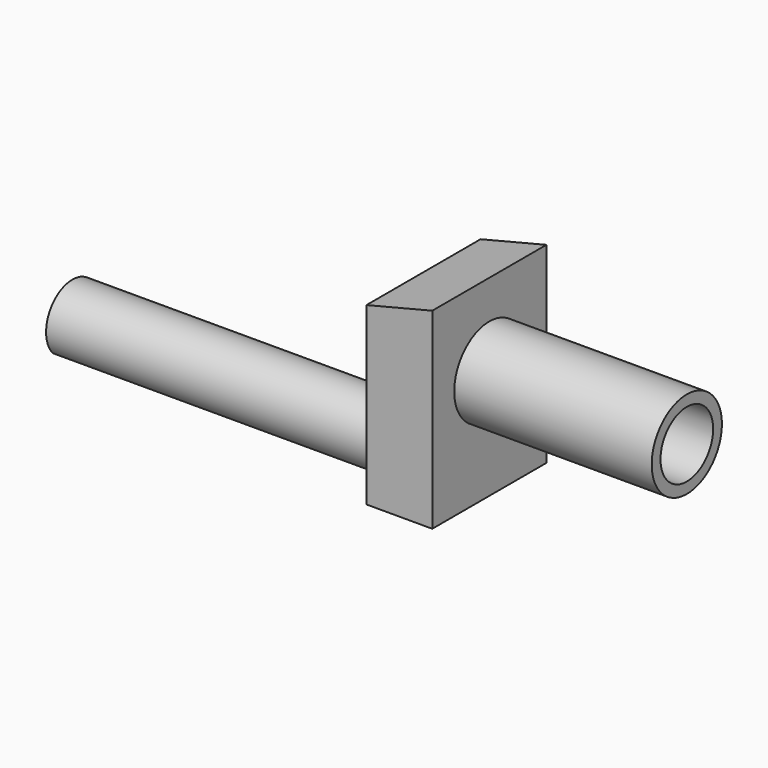
from build123d import *

# Parameters (mm, degrees)
F1_DEPTH  = 20.6375
F2_R      = 9.525
F3_DEPTH  = 50.8
F5_DEPTH  = 127
F7_DEPTH  = 41.276
F8_W      = 41.275
F8_H      = 69.85
F8_R      = 12.7
F9_DEPTH  = 57.15
F10_W     = 25.4
F10_H     = 32.7966427431
F11_DEPTH = 34.926


# Not quite as in the source:
# - a feature names something its author has since deleted; it is built from what else it names


with BuildPart() as f1:
    # F0 (on Front) → F1 (new body, symmetric)
    with BuildSketch(Plane.XZ):
        Polygon((-101.6, -34.925), (101.6, -34.925), (101.6, 34.925), (-101.6, -15.875), align=None)
    extrude(amount=F1_DEPTH, both=True)

    # F2 (on face) → F3 (cut)
    with BuildSketch(Plane.YZ.offset(101.6)):
        with Locations((0, -3.175)):
            Circle(F2_R)
    extrude(amount=-F3_DEPTH, mode=Mode.SUBTRACT)

    # F4 (on face) → F5 (cut)
    with BuildSketch(Plane(origin=(-101.6, 0, 0), x_dir=(0, -1, 0), z_dir=(-1, 0, 0))):
        with BuildLine():
            ThreePointArc((-7.0995158286, -34.925), (0, -19.05), (7.0995158286, -34.925))
            Line((7.0995158286, -34.925), (20.6375, -34.925))
            Line((20.6375, -34.925), (20.6375, -15.875))
            Line((20.6375, -15.875), (-20.6375, -15.875))
            Line((-20.6375, -15.875), (-20.6375, -34.925))
            Line((-20.6375, -34.925), (-7.0995158286, -34.925))
        make_face()
    extrude(amount=-F5_DEPTH, mode=Mode.SUBTRACT)

    # F6 (on face) → F7 (cut, through all)
    with BuildSketch(Plane(origin=(0, 20.6375, 0), x_dir=(-1, 0, 0), z_dir=(0, 1, 0))):
        Polygon((-25.4, 15.875), (-25.4, -15.875), (101.6, -15.875), align=None)
    extrude(amount=-F7_DEPTH, mode=Mode.SUBTRACT)

    # F8 (on face) → F9 (cut)
    with BuildSketch(Plane.YZ.offset(101.6)):
        Rectangle(F8_W, F8_H)
        with Locations((0, -3.175)):
            Circle(F8_R, mode=Mode.SUBTRACT)
    extrude(amount=-F9_DEPTH, mode=Mode.SUBTRACT)

    # F10 (on Top) → F11 (cut, through all)
    with BuildSketch(Plane.XY):
        with Locations((-88.9, -1.6974383034)):
            Rectangle(F10_W, F10_H)
    extrude(amount=-F11_DEPTH, mode=Mode.SUBTRACT)


solid = f1.part
